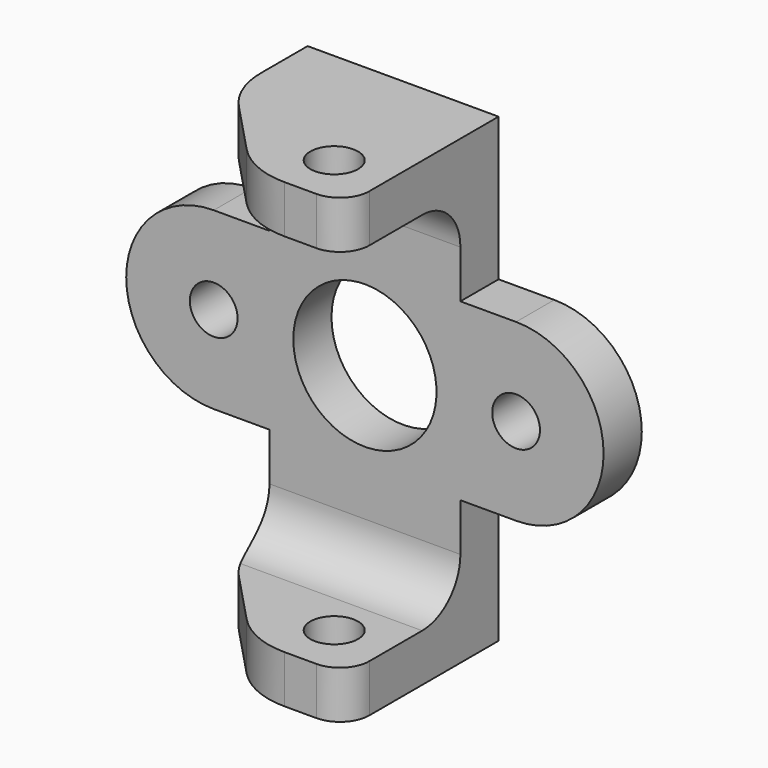
from build123d import *

# Parameters (mm, degrees)
F0_R     = 1.5
F0_R_2   = 4.5
F1_DEPTH = 3
F2_W     = 12
F2_H     = 29
F3_DEPTH = 3
F4_R     = 1.5
F5_DEPTH = 3
F7_R     = 3
F8_R     = 4.5
F9_DEPTH = 3


with BuildPart() as f1:
    # F0 (on Front) → F1 (new body)
    with BuildSketch(Plane.XZ):
        with BuildLine():
            Line((0, -5.5), (9.5, -5.5))
            ThreePointArc((9.5, -5.5), (15, 0), (9.5, 5.5))
            Line((9.5, 5.5), (0, 5.5))
            Line((0, 5.5), (-9.5, 5.5))
            ThreePointArc((-9.5, 5.5), (-15, 0), (-9.5, -5.5))
            Line((-9.5, -5.5), (0, -5.5))
        make_face()
        with Locations((-9.5, 0)):
            Circle(F0_R, mode=Mode.SUBTRACT)
        Circle(F0_R_2, mode=Mode.SUBTRACT)
        with Locations((9.5, 0)):
            Circle(F0_R, mode=Mode.SUBTRACT)
    extrude(amount=F1_DEPTH)

    # F2 (on face) → F3 (join)
    with BuildSketch(Plane.XZ.offset(3)):
        Rectangle(F2_W, F2_H)
    extrude(amount=-F3_DEPTH)

    # F4 (on face) → F5 (join)
    with BuildSketch(Plane(origin=(0, 0, -14.5), x_dir=(1, 0, 0), z_dir=(0, 0, -1))):
        with BuildLine():
            Line((-6, 0), (6, 0))
            Line((6, 0), (6, 10.1512318682))
            ThreePointArc((6, 10.1512318682), (5.458508351, 11.458508351), (4.1512318682, 12))
            Line((4.1512318682, 12), (2.1505740618, 12))
            ThreePointArc((2.1505740618, 12), (0.1749902584, 11.5931545408), (-1.4790906252, 10.4388274542))
            Line((-1.4790906252, 10.4388274542), (-4.629664687, 7.11341274))
            ThreePointArc((-4.629664687, 7.11341274), (-5.6447994271, 5.5254873044), (-6, 3.6745852858))
            Line((-6, 3.6745852858), (-6, 0))
        make_face()
        with Locations((2.5998784695, 8.662102744)):
            Circle(F4_R, mode=Mode.SUBTRACT)
    extrude(amount=-F5_DEPTH)

    # F6: F1 across plane


with BuildPart() as f1_1:
    add(f1.part)
    add(f1.part.mirror(Plane.XY))

    # F7
    f7_edges = [f1_1.edges().sort_by_distance(p)[0] for p in [
        (0, -3, 11.5),
        (0, -3, -11.5),
    ]]
    fillet(f7_edges, radius=F7_R)

    # F8 (on face) → F9 (cut, through all)
    with BuildSketch(Plane(origin=(0, 0, 0), x_dir=(-1, 0, 0), z_dir=(0, 1, 0))):
        Circle(F8_R)
    extrude(amount=-F9_DEPTH, mode=Mode.SUBTRACT)


solid = f1_1.part
